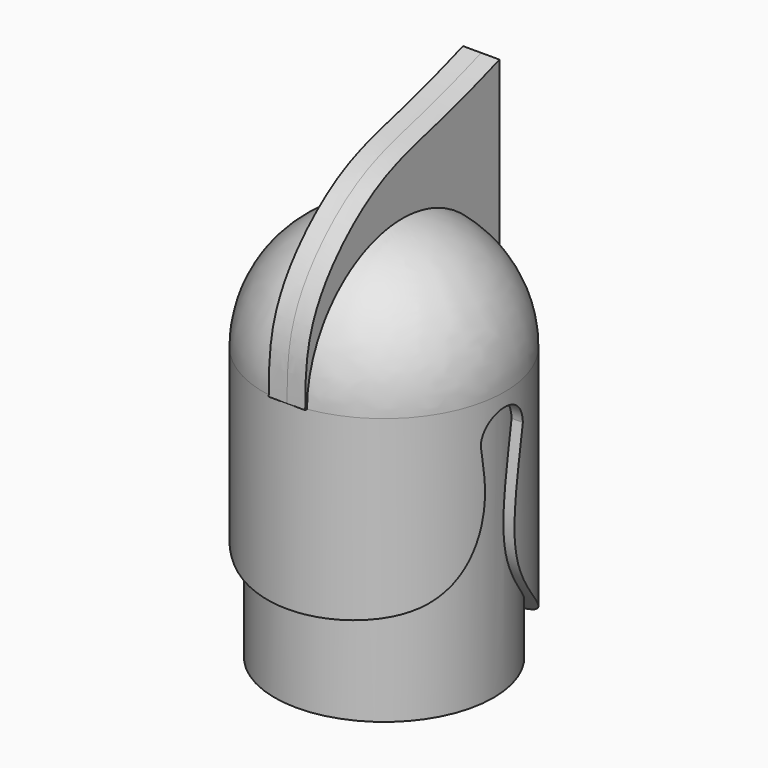
from build123d import *

# Parameters (mm, degrees)
F3_DEPTH = 78.232
F5_DEPTH = 76.708
F7_DEPTH = 8.382


with BuildPart() as f1:
    # F0 (on Front) → F1 (revolve)
    with BuildSketch(Plane.XZ):
        with BuildLine():
            ThreePointArc((-0.0698173458, 55.5173469571), (-39.2813999528, 39.2320316243), (-55.5173908575, 0))
            Line((-55.5173908575, 0), (-55.5173908575, -139.9010568857))
            Line((-55.5173908575, -139.9010568857), (-50.3665891177, -139.9010568857))
            Line((-50.3665891177, -139.9010568857), (-50.3665891177, 0))
            ThreePointArc((-50.3665891177, 0), (-35.6392323214, 35.5898639909), (-0.0698173458, 50.3665407278))
            Line((-0.0698173458, 50.3665407278), (-0.0698173458, 55.5173469571))
        make_face()
    revolve(axis=Axis((-0.0698173458, 0, -42.1918549643), (0, 0, -1)))

    # F2 (on Front) → F3 (cut)
    with BuildSketch(Plane.XZ):
        with BuildLine():
            Line((7.5376802124, -48.7698412978), (0, -53.0028641224))
            Line((0, -53.0028641224), (-7.5376802124, -48.7698412978))
            Line((-7.5376802124, -48.7698412978), (-7.5376802124, -13.3147090673))
            add(Edge.make_bspline(
                [(-7.5376802124, -13.3147090673), (-10.6544717683, -12.1152898726), (-17.0466209172, -9.6554313138), (-29.2889640988, -10.2190826436), (-38.3318119855, -22.0312493196), (-44.7023774494, -32.2462858121), (-32.6443109339, -30.6446020866), (-25.4389418575, -29.6875064884)],
                knots=[0, 0, 0, 0, 0.1858869155, 0.381230784, 0.6097084328, 0.766778962, 1, 1, 1, 1], degree=3))
            Line((-25.4389418575, -29.6875064884), (-25.1471186057, -139.449729957))
            Line((-25.1471186057, -139.449729957), (-25.1471186057, -147.9396272018))
            Line((-25.1471186057, -147.9396272018), (25.1700459273, -147.805849677))
            Line((25.1700459273, -147.805849677), (25.1474741186, -139.3160124436))
            Line((25.1474741186, -139.3160124436), (25.4389418575, -29.6875064884))
            add(Edge.make_bspline(
                [(7.5376802124, -13.3147090673), (10.6544717683, -12.1152898726), (17.0466209172, -9.6554313138), (29.2889640988, -10.2190826436), (38.3318119855, -22.0312493196), (44.7023774494, -32.2462858121), (32.6443109339, -30.6446020866), (25.4389418575, -29.6875064884)],
                knots=[0, 0, 0, 0, 0.1858869155, 0.381230784, 0.6097084328, 0.766778962, 1, 1, 1, 1], degree=3))
            Line((7.5376802124, -13.3147090673), (7.5376802124, -48.7698412978))
        make_face()
    extrude(amount=-F3_DEPTH, mode=Mode.SUBTRACT)

    # F4 (on Right) → F5 (cut, symmetric)
    with BuildSketch(Plane.YZ):
        with BuildLine():
            add(Edge.make_bspline(
                [(12.1212325205, -17.766580238), (7.9757607956, -36.6438234259), (0.5209855272, -70.519007332), (25.7770894943, -97.3501854501), (41.6857298717, -110.939256132), (49.5449826121, -117.6521554589)],
                knots=[0, 0, 0, 0, 0.3890830913, 0.6982091981, 1, 1, 1, 1], degree=3))
            ThreePointArc((12.1212325205, -17.766580238), (0.2853212514, -6.1320097846), (-12.0846225247, -17.1971133169))
            add(Edge.make_bspline(
                [(-12.0846225247, -17.1971133169), (-11.867728969, -18.8822483457), (-11.6508517517, -20.5673831054), (-11.4435163526, -22.2865332031)],
                knots=[0, 0, 0, 0, 0.1306441435, 0.1306441435, 0.1306441435, 0.1306441435], degree=3))
            Line((-11.4435163526, -22.2865332031), (-11.3662809338, -22.7782038834))
            add(Edge.make_bspline(
                [(-10.1156651322, -38.743025822), (-9.9494934772, -33.2704634022), (-10.6578872055, -28.0243336428), (-11.3662809338, -22.7782038834)],
                knots=[0.7988740642, 0.7988740642, 0.7988740642, 0.7988740642, 1, 1, 1, 1], degree=3))
            add(Edge.make_bspline(
                [(-55.9491626918, -83.4509804845), (-47.7624356842, -81.8508821411), (-31.8258782431, -78.7360770258), (-15.1130072731, -62.8612092803), (-10.5650326322, -47.2975358408), (-10.1416441707, -39.5985983927), (-10.1156651322, -38.743025822)],
                knots=[0, 0, 0, 0, 0.2659687103, 0.5177436141, 0.7674303235, 0.7988740642, 0.7988740642, 0.7988740642, 0.7988740642], degree=3))
            Line((-55.9491626918, -83.4509804845), (-55.9491626918, -146.6366350651))
            Line((-55.9491626918, -146.6366350651), (49.5449826121, -146.6366350651))
            Line((49.5449826121, -146.6366350651), (49.5449826121, -138.8599425554))
            Line((49.5449826121, -138.8599425554), (49.5449826121, -117.6521554589))
        make_face()
    extrude(amount=F5_DEPTH, both=True, mode=Mode.SUBTRACT)

    # F6 (on Right) → F7 (join, symmetric)
    with BuildSketch(Plane.YZ):
        with BuildLine():
            Line((51.3022430241, 0), (55.7309389114, 0))
            Line((55.7309389114, 0), (55.7309389114, 96.4915975928))
            add(Edge.make_bspline(
                [(-55.8152869344, 0), (-55.7341075294, 8.6070727552), (-55.5693222875, 26.0784814912), (-43.6280408785, 51.3808987642), (-13.3631377226, 77.8522856682), (24.2078567943, 85.5107411936), (45.4746019366, 92.9188706912), (55.7309389114, 96.4915975928)],
                knots=[0, 0, 0, 0, 0.1776302277, 0.3605697779, 0.5798025952, 0.7973509274, 1, 1, 1, 1], degree=3))
            Line((-55.8152869344, 0), (-51.3022430241, 0))
            ThreePointArc((-51.3022430241, 0), (0, 51.3022430241), (51.3022430241, 0))
        make_face()
    extrude(amount=F7_DEPTH, both=True)

    # F8 (on Right) → F9 (revolve)
    with BuildSketch(Plane.YZ):
        with BuildLine():
            Line((0, -123.9440590143), (0, 50.3170703726))
            ThreePointArc((0, 50.3170703726), (-35.5795416699, 35.5795416699), (-50.3170703726, 0))
            Line((-50.3170703726, 0), (-50.3170703726, -125.3333687782))
            Line((-50.3170703726, -125.3333687782), (0, -125.3333687782))
            Line((0, -125.3333687782), (0, -123.9440590143))
        make_face()
    revolve(axis=Axis((0, 0, -36.7921870202), (0, 0, -1)))


solid = f1.part
